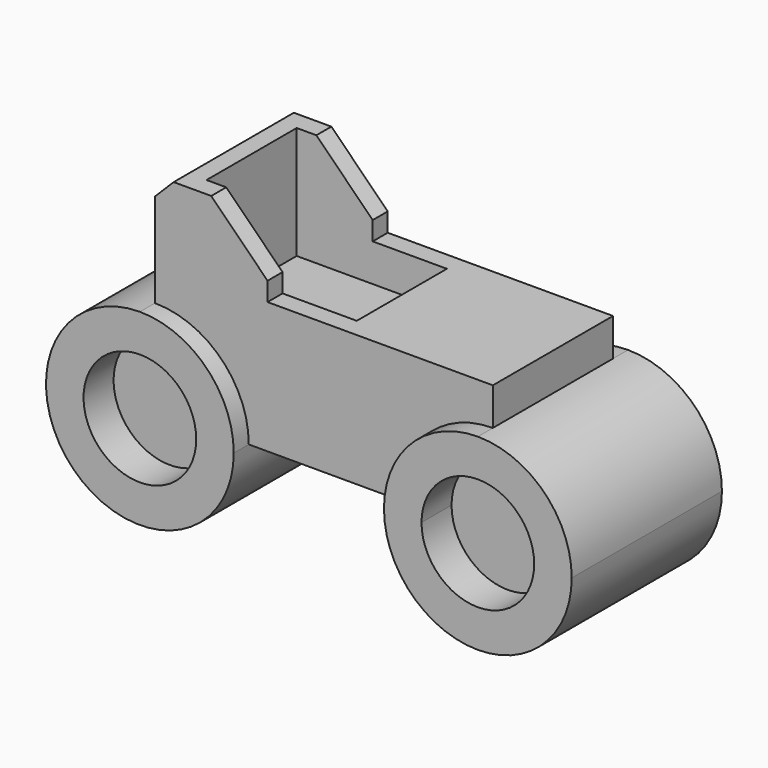
from build123d import *

# Parameters (mm, degrees)
F1_DEPTH = 20
F2_DEPTH = 25
F3_DEPTH = 15
F5_START = 7.5
F5_DEPTH = 30


with BuildPart() as f1:
    # F0 (on Front) → F1 (new body, symmetric)
    with BuildSketch(Plane.XZ):
        with BuildLine():
            ThreePointArc((-45, 7.5), (-27.32233, 0.17767), (-20, -17.5))
            Line((-20, -17.5), (20, -17.5))
            ThreePointArc((20, -17.5), (27.32233, 0.17767), (45, 7.5))
            Line((45, 7.5), (45, 17.5))
            Line((45, 17.5), (-15, 17.5))
            Line((-15, 17.5), (-45, 17.5))
            Line((-45, 17.5), (-45, 7.5))
        make_face()
        Polygon((-45, 32.5), (-45, 17.5), (-15, 17.5), (-15, 22.5), (-30, 37.5), (-40, 37.5), align=None)
    extrude(amount=F1_DEPTH, both=True)

    # F0 (on Front) → F2 (join, symmetric)
    with BuildSketch(Plane.XZ):
        with BuildLine():
            Line((30, -17.5), (20, -17.5))
            ThreePointArc((20, -17.5), (45, -42.5), (70, -17.5))
            ThreePointArc((70, -17.5), (62.67767, 0.17767), (45, 7.5))
            Line((45, 7.5), (45, -2.5))
            ThreePointArc((45, -2.5), (55.606602, -6.893398), (60, -17.5))
            ThreePointArc((60, -17.5), (45, -32.5), (30, -17.5))
        make_face()
        with BuildLine():
            ThreePointArc((45, 7.5), (27.32233, 0.17767), (20, -17.5))
            Line((20, -17.5), (30, -17.5))
            ThreePointArc((30, -17.5), (34.393398, -6.893398), (45, -2.5))
            Line((45, -2.5), (45, 7.5))
        make_face()
        with BuildLine():
            ThreePointArc((-45, 7.5), (-62.67767, -35.17767), (-20, -17.5))
            Line((-20, -17.5), (-30, -17.5))
            ThreePointArc((-30, -17.5), (-55.606602, -28.106602), (-45, -2.5))
            Line((-45, -2.5), (-45, 7.5))
        make_face()
        with BuildLine():
            Line((-30, -17.5), (-20, -17.5))
            ThreePointArc((-20, -17.5), (-27.32233, 0.17767), (-45, 7.5))
            Line((-45, 7.5), (-45, -2.5))
            ThreePointArc((-45, -2.5), (-34.393398, -6.893398), (-30, -17.5))
        make_face()
    extrude(amount=F2_DEPTH, both=True)

    # F0 (on Front) → F3 (join, symmetric)
    with BuildSketch(Plane.XZ):
        with BuildLine():
            Line((45, -17.5), (30, -17.5))
            ThreePointArc((30, -17.5), (45, -32.5), (60, -17.5))
            ThreePointArc((60, -17.5), (55.606602, -6.893398), (45, -2.5))
            Line((45, -2.5), (45, -17.5))
        make_face()
        with BuildLine():
            ThreePointArc((45, -2.5), (34.393398, -6.893398), (30, -17.5))
            Line((30, -17.5), (45, -17.5))
            Line((45, -17.5), (45, -2.5))
        make_face()
        with BuildLine():
            ThreePointArc((-45, -2.5), (-55.606602, -28.106602), (-30, -17.5))
            Line((-30, -17.5), (-45, -17.5))
            Line((-45, -17.5), (-45, -2.5))
        make_face()
        with BuildLine():
            Line((-45, -17.5), (-30, -17.5))
            ThreePointArc((-30, -17.5), (-34.393398, -6.893398), (-45, -2.5))
            Line((-45, -2.5), (-45, -17.5))
        make_face()
    extrude(amount=F3_DEPTH, both=True)

    # F4 (on Top) → F5 (cut)
    with BuildSketch(Plane.XY.offset(F5_START)):
        Polygon((-35.244276, 15), (-35.244276, 0), (-35.244276, -15), (4.755724, -15), (4.755724, 15), align=None)
    extrude(amount=F5_DEPTH, mode=Mode.SUBTRACT)


solid = f1.part
